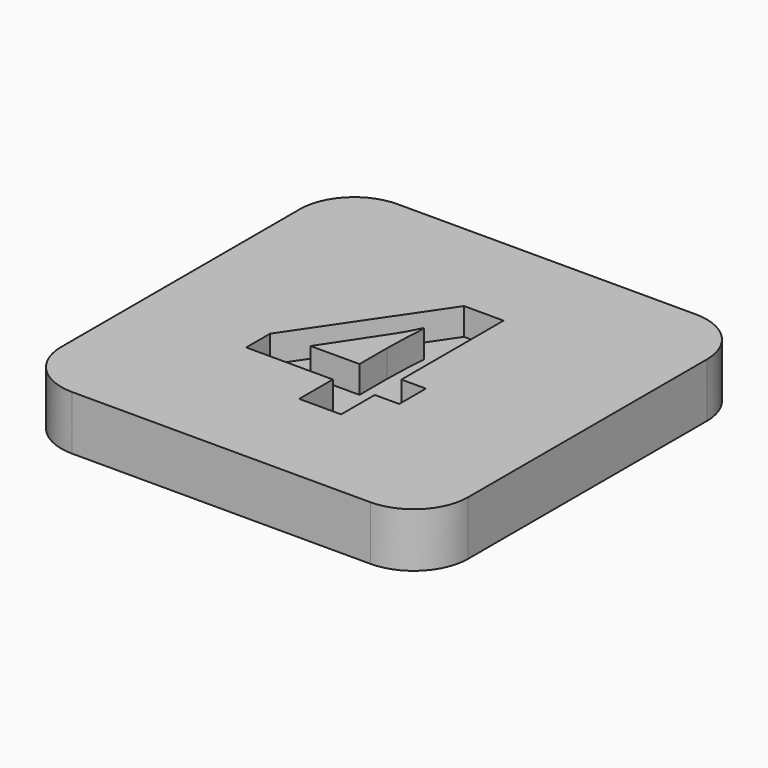
from build123d import *

# Parameters (mm, degrees)
F0_W         = 38.1
F0_H         = 38.1
F1_DEPTH     = 5.08
F2_TEXT_SIZE = 26.6290322581
F3_DEPTH     = 2.54
F4_R         = 5.08


# Not quite as in the source:
# - Text() gives the source's letters only with a copy of the font that has no kerning and outlines rounded to 1/6400 em; it was checked with that copy


with BuildPart() as f1:
    # F0 (on Top) → F1 (new body)
    with BuildSketch(Plane.XY):
        Rectangle(F0_W, F0_H)
    extrude(amount=F1_DEPTH)

    # F2 (on face) → F3 (cut)
    with BuildSketch(Plane.XY.offset(5.08)):
        with Locations((-8.89, -9.525)):
            Text('4', F2_TEXT_SIZE, font='Open Sans', font_style=FontStyle.BOLD, text_align=(TextAlign.LEFT, TextAlign.BOTTOM))
    extrude(amount=-F3_DEPTH, mode=Mode.SUBTRACT)

    # F4
    f4_edges = [f1.edges().sort_by_distance(p)[0] for p in [
        (-19.05, -19.05, 2.54),
        (19.05, -19.05, 2.54),
        (19.05, 19.05, 2.54),
        (-19.05, 19.05, 2.54),
    ]]
    fillet(f4_edges, radius=F4_R)


solid = f1.part
